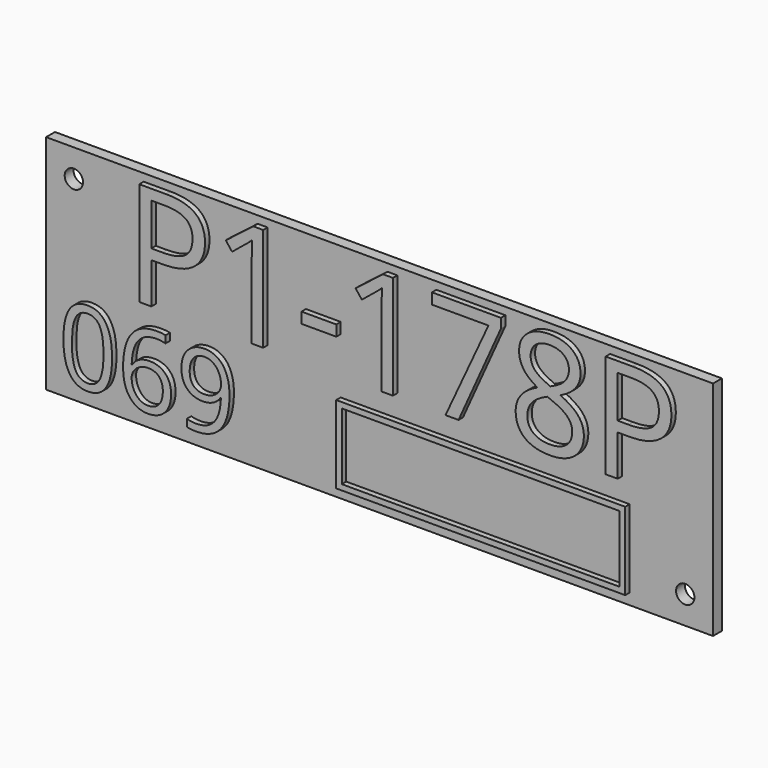
from build123d import *

# Parameters (mm, degrees)
F0_W         = 120
F0_H         = 40
F1_DEPTH     = 2
F3_D         = 3.3
F4_TEXT_SIZE = 26.1352499183
F5_DEPTH     = 1
F6_TEXT_SIZE = 18.5356140827
F7_DEPTH     = 1
F8_W         = 52
F8_H         = 14
F8_W_2       = 49.99999962
F8_H_2       = 11.99999962
F9_DEPTH     = 1


# Not quite as in the source:
# - Text() gives the source's letters only with a copy of the font that has no kerning and outlines rounded to 1/6400 em; it was checked with that copy


with BuildPart() as f1:
    # F0 (on Front) → F1 (new body)
    with BuildSketch(Plane.XZ):
        Rectangle(F0_W, F0_H)
    extrude(amount=F1_DEPTH)

    # F3 (through all)
    with Locations(Plane.XZ.offset(2)):
        with Locations((-55, 15), (55, -15)):
            Hole(F3_D / 2)

    # F4 (on face) → F5 (join)
    with BuildSketch(Plane.XZ.offset(2)):
        with Locations((-45, 0)):
            Text('P1-178P', F4_TEXT_SIZE, font='Open Sans', text_align=(TextAlign.LEFT, TextAlign.BOTTOM))
    extrude(amount=F5_DEPTH)

    # F6 (on face) → F7 (join)
    with BuildSketch(Plane.XZ.offset(2)):
        with Locations((-57, -17)):
            Text('069', F6_TEXT_SIZE, font='Open Sans', text_align=(TextAlign.LEFT, TextAlign.BOTTOM))
    extrude(amount=F7_DEPTH)

    # F8 (on face) → F9 (join)
    with BuildSketch(Plane.XZ.offset(2)):
        with Locations((19, -11)):
            Rectangle(F8_W, F8_H)
        with Locations((19, -11)):
            Rectangle(F8_W_2, F8_H_2, mode=Mode.SUBTRACT)
    extrude(amount=F9_DEPTH)


solid = f1.part
